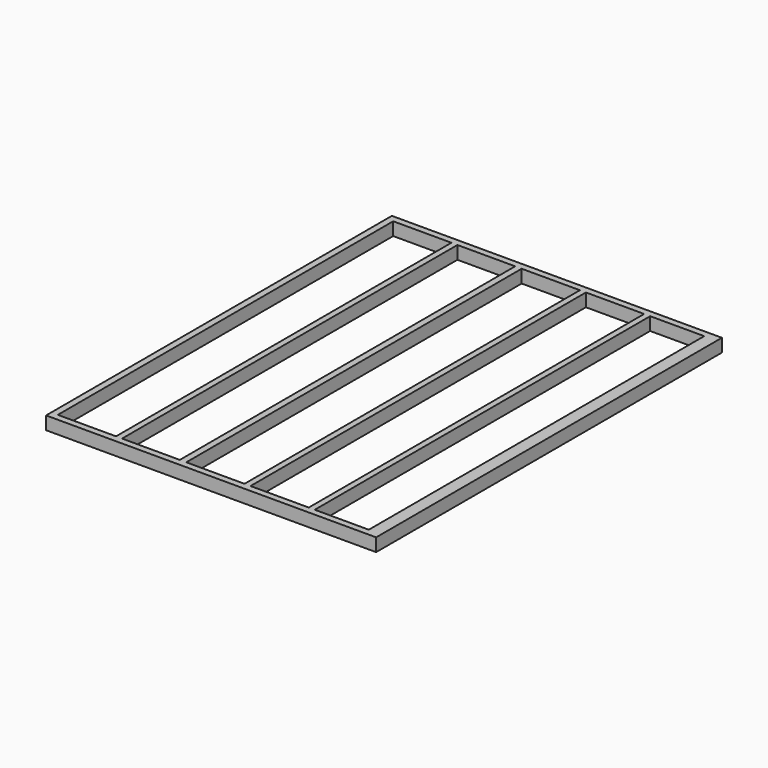
from build123d import *

# Parameters (mm, degrees)
F0_W     = 2087.5752
F0_H     = 2733.7512
F0_W_2   = 38.1
F0_H_2   = 2651.4552
F0_W_3   = 37.9984
F0_W_4   = 41.148
F1_DEPTH = 82.55


# Not quite as in the source:
# - a feature names something its author has since deleted; it is built from what else it names


with BuildPart() as f1:
    # F0 (on Top) → F1 (new body)
    with BuildSketch(Plane.XY):
        Rectangle(F0_W, F0_H)
        Polygon((1002.6396, 1325.7276), (1002.6396, -1325.7276), (964.5396, -1325.7276), (622.7572, -1325.7276), (584.7588, -1325.7276), (216.4588, -1325.7276), (178.3588, -1325.7276), (-189.8396, -1325.7276), (-230.9876, -1325.7276), (-596.138, -1325.7276), (-634.238, -1325.7276), (-1002.4364, -1325.7276), (-1002.4364, 1325.7276), (-634.238, 1325.7276), (-596.138, 1325.7276), (-230.9876, 1325.7276), (-189.8396, 1325.7276), (178.3588, 1325.7276), (216.4588, 1325.7276), (584.7588, 1325.7276), (622.7572, 1325.7276), (964.5396, 1325.7276), align=None, mode=Mode.SUBTRACT)
        with Locations((983.5896, 0)):
            Rectangle(F0_W_2, F0_H_2)
        with Locations((603.758, 0)):
            Rectangle(F0_W_3, F0_H_2)
        with Locations((197.4088, 0)):
            Rectangle(F0_W_2, F0_H_2)
        with Locations((-210.4136, 0)):
            Rectangle(F0_W_4, F0_H_2)
        with Locations((-615.188, 0)):
            Rectangle(F0_W_2, F0_H_2)
    extrude(amount=F1_DEPTH)


solid = f1.part
